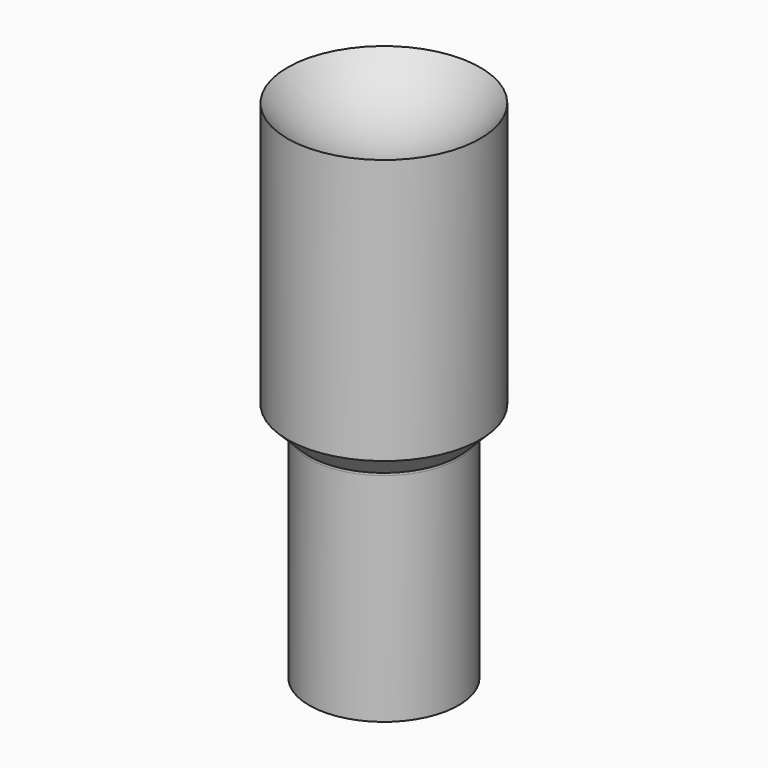
from build123d import *

# Parameters (mm, degrees)
F0_W        = 3.1
F0_H        = 9
F2_S5_R     = 3.1
F2_T6_DEPTH = 7


# Not quite as in the source:
# - a fillet or chamfer that OpenCascade refuses, or shapes differently, is made with other operations: its cross-section is extruded or revolved along the edge and cut away or added


with BuildPart() as f1:
    # F0 (on Front) → F1 (revolve)
    with BuildSketch(Plane.XZ):
        with Locations((-1.55, -4.5)):
            Rectangle(F0_W, F0_H)
        with BuildLine():
            Line((0, 0), (0, 10))
            ThreePointArc((0, 10), (-2.2360679775, 10.527864045), (-4, 12))
            Line((-4, 12), (-4, 0))
            Line((-4, 0), (-3.1, 0))
            Line((-3.1, 0), (0, 0))
        make_face()
    revolve(axis=Axis((0, 0, 1.5), (0, 0, -1)))

    # F2: chamfer of 1 on 1 edges, made by hand


with BuildPart() as f2_tool2:
    # F2_s3 → F2_t4 (revolve)
    with BuildSketch(Plane.XZ):
        Polygon((-4, 1), (-3, 0), (-4, 0), align=None)
    revolve(axis=Axis((0, 0, 0), (0, 0, -1)))

    # F2_s5 → F2_t6 (cut, symmetric)
    with BuildSketch(Plane.XY.offset(0.5)):
        Circle(F2_S5_R)
    extrude(amount=F2_T6_DEPTH, both=True, mode=Mode.SUBTRACT)


with BuildPart() as f1_1:
    add(f1.part)

    # F2_t1: cut F2_tool2
    add(f2_tool2.part, mode=Mode.SUBTRACT)


solid = f1_1.part
